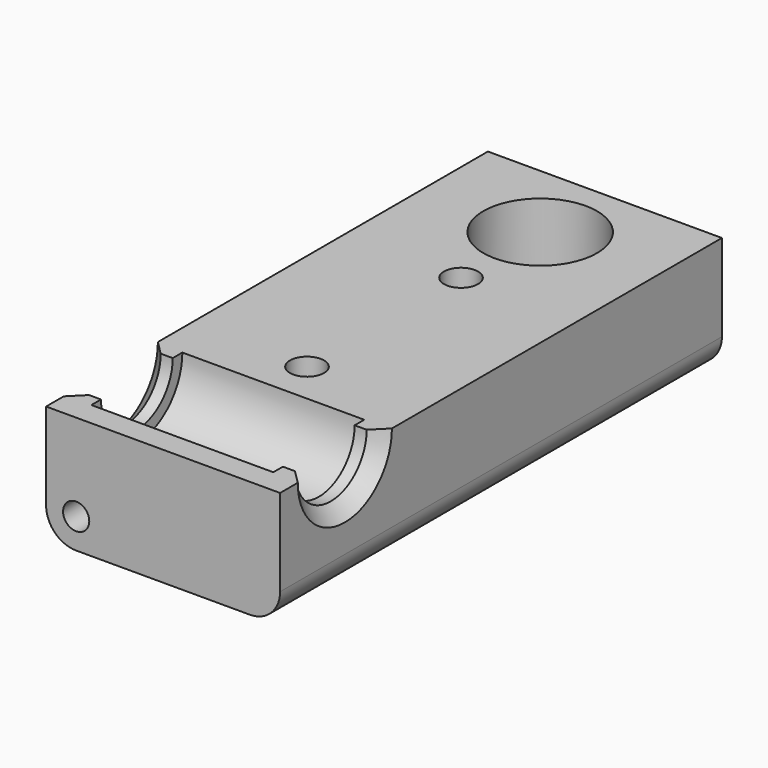
from build123d import *

# Parameters (mm, degrees)
F0_W      = 30.8750208
F0_H      = 72.8625058
F0_R      = 2.2479
F0_R_2    = 5.9124977
F1_DEPTH  = 3.437509
F2_W      = 30.8750208
F2_H      = 72.8625058
F2_R      = 2.2479
F2_R_2    = 7.5
F3_DEPTH  = 12
F4_W      = 24
F4_H      = 15
F5_DEPTH  = 7.5
F6_R      = 7.49999
F8_DEPTH  = 30.8750208
F9_R      = 3.96875
F10_DEPTH = 9.0875104
F11_R     = 3.96875
F12_R     = 1.7272
F13_DEPTH = 6.35
F14_SIZE  = 1.850009


# Not quite as in the source:
# - a fillet or chamfer is up to 0.001 mm smaller than in the source, because OpenCascade refuses the exact size


with BuildPart() as f1:
    # F0 (on Top) → F1 (new body)
    with BuildSketch(Plane.XY):
        with Locations((15.4375104, -36.4312529)):
            Rectangle(F0_W, F0_H)
        with Locations((15.4375104, -49.1312477)):
            Circle(F0_R, mode=Mode.SUBTRACT)
        with Locations((15.4375104, -23.7312477)):
            Circle(F0_R, mode=Mode.SUBTRACT)
        with Locations((15.4375104, -10.6749977)):
            Circle(F0_R_2, mode=Mode.SUBTRACT)
    extrude(amount=F1_DEPTH)

    # F2 (on face) → F3 (join)
    with BuildSketch(Plane.XY.offset(3.437509)):
        with Locations((15.4375104, -36.4312529)):
            Rectangle(F2_W, F2_H)
        with Locations((15.4375104, -49.1312477)):
            Circle(F2_R, mode=Mode.SUBTRACT)
        with Locations((15.4375104, -23.7312477)):
            Circle(F2_R, mode=Mode.SUBTRACT)
        with Locations((15.4375104, -10.6749977)):
            Circle(F2_R_2, mode=Mode.SUBTRACT)
    extrude(amount=F3_DEPTH)

    # F4 (on face) → F5 (cut)
    with BuildSketch(Plane.XY.offset(15.437509)):
        with Locations((15.4375104, -62.1875058)):
            Rectangle(F4_W, F4_H)
    extrude(amount=-F5_DEPTH, mode=Mode.SUBTRACT)

    # F6 (radius 7.5 in the source; OpenCascade refuses exactly that, so slightly less here)
    f6_edges = [f1.edges().sort_by_distance(p)[0] for p in [
        (15.43751, -54.687506, 7.937509),
        (15.43751, -69.687506, 7.937509),
    ]]
    fillet(f6_edges, radius=F6_R)

    # F7 (on face) → F8 (cut, through all)
    with BuildSketch(Plane(origin=(0, 0, 0), x_dir=(0, -1, 0), z_dir=(-1, 0, 0))):
        with BuildLine():
            Line((68.1000035, 15.437509), (56.2750081, 15.437509))
            ThreePointArc((56.2750081, 15.437509), (62.1875058, 9.5250113), (68.1000035, 15.437509))
        make_face()
    extrude(amount=-F8_DEPTH, mode=Mode.SUBTRACT)

    # F9 (on face) → F10 (cut)
    with BuildSketch(Plane(origin=(0, 0, 0), x_dir=(1, 0, 0), z_dir=(0, 0, -1))):
        with Locations((15.4375104, 23.7312477)):
            Circle(F9_R)
        with Locations((15.4375104, 49.1312477)):
            Circle(F9_R)
    extrude(amount=-F10_DEPTH, mode=Mode.SUBTRACT)

    # F11
    f11_edges = [f1.edges().sort_by_distance(p)[0] for p in [
        (0, -36.431253, 0),
        (30.875021, -36.431253, 0),
    ]]
    fillet(f11_edges, radius=F11_R)

    # F12 (on face) → F13 (cut)
    with BuildSketch(Plane.XZ.offset(72.8625058)):
        with Locations((3.96875, 3.96875)):
            Circle(F12_R)
    extrude(amount=-F13_DEPTH, mode=Mode.SUBTRACT)

    # F14
    f14_edges = [f1.edges().sort_by_distance(p)[0] for p in [
        (9.525013, -10.674998, 0),
        (30.875021, -62.187506, 9.525011),
        (0, -62.187506, 9.525011),
    ]]
    chamfer(f14_edges, length=F14_SIZE)


solid = f1.part
